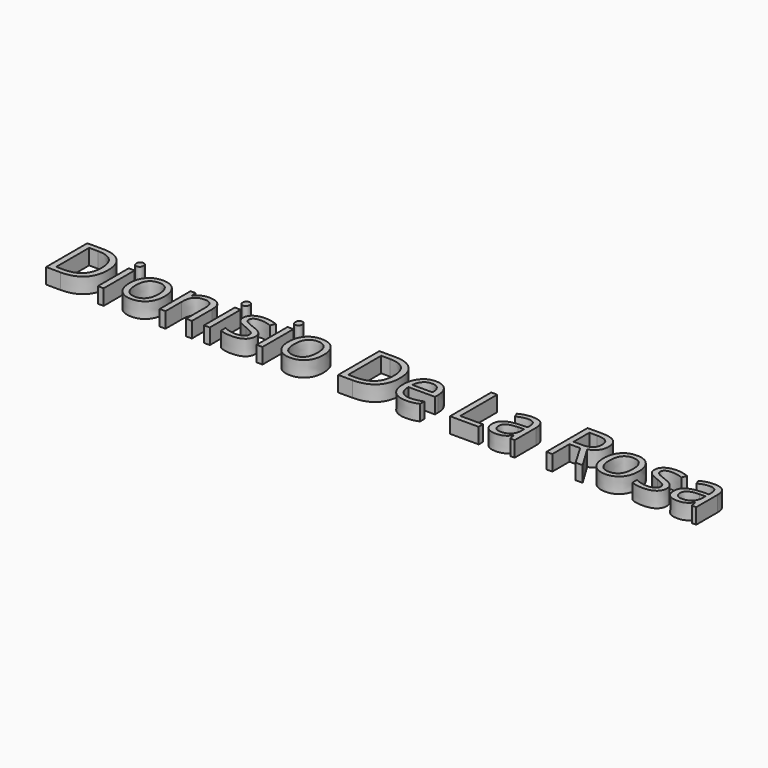
from build123d import *

# Parameters (mm, degrees)
F0_TEXT_SIZE = 118.2675620334
F1_DEPTH     = 25.4


# Not quite as in the source:
# - Text() gives the source's letters only with a copy of the font that has no kerning and outlines rounded to 1/6400 em; it was checked with that copy


with BuildPart() as f1:
    # F0 (on Top) → F1 (new body)
    with BuildSketch(Plane.XY):
        with Locations((-392.1324945986, -29.1586555541)):
            Text('Dionisio De La Rosa', F0_TEXT_SIZE, font='Open Sans', text_align=(TextAlign.LEFT, TextAlign.BOTTOM))
    extrude(amount=F1_DEPTH)


solid = f1.part
